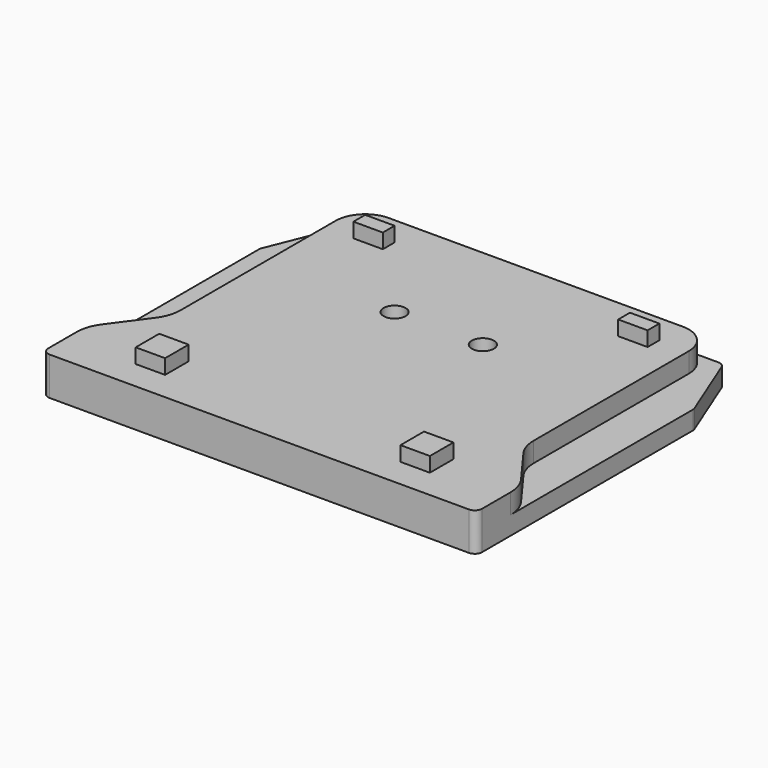
from build123d import *

# Parameters (mm, degrees)
F1_DEPTH      = 2.5
F3_DEPTH      = 2.7
F4_R          = 1
F5_R          = 5
F6_W          = 4
F6_H          = 2
F6_H_2        = 4
F7_DEPTH      = 2
F8_R          = 1.5
F9_DEPTH      = 6
F10_R         = 2.5
F11_DEPTH     = 2.5
F12_S5_R      = 1.5
F12_T6_DEPTH  = 5
F12_S11_R     = 1.5
F12_T12_DEPTH = 5


# Not quite as in the source:
# - a fillet or chamfer that OpenCascade refuses, or shapes differently, is made with other operations: its cross-section is extruded or revolved along the edge and cut away or added


with BuildPart() as f1:
    # F0 (on Top) → F1 (new body)
    with BuildSketch(Plane.XY):
        Polygon((55, 0), (4, 0), (0, -10), (0, -47), (59, -47), (59, -10), align=None)
    extrude(amount=F1_DEPTH)

    # F2 (on face) → F3 (join)
    with BuildSketch(Plane.XY.offset(2.5)):
        with BuildLine():
            Line((0, -39.5), (0, -47))
            Line((0, -47), (59, -47))
            Line((59, -47), (59, -39.5))
            Line((59, -39.5), (53.5, -32))
            Line((53.5, -32), (53.5, -4))
            ThreePointArc((53.5, -4), (52.3284271247, -1.1715728753), (49.5, 0))
            Line((49.5, 0), (9.5, 0))
            ThreePointArc((9.5, 0), (6.6715728753, -1.1715728753), (5.5, -4))
            Line((5.5, -4), (5.5, -32))
            Line((5.5, -32), (0, -39.5))
        make_face()
    extrude(amount=F3_DEPTH)

    # F4
    f4_edges = [f1.edges().sort_by_distance(p)[0] for p in [
        (0, -47, 2.6),
        (59, -47, 2.6),
        (4, 0, 1.25),
        (55, 0, 1.25),
        (59, -10, 1.25),
        (0, -10, 1.25),
    ]]
    fillet(f4_edges, radius=F4_R)

    # F5
    f5_edges = [f1.edges().sort_by_distance(p)[0] for p in [
        (0, -39.5, 3.85),
        (59, -39.5, 3.85),
        (53.5, -32, 3.85),
        (5.5, -32, 3.85),
    ]]
    fillet(f5_edges, radius=F5_R)

    # F6 (on face) → F7 (join)
    with BuildSketch(Plane.XY.offset(5.2)):
        with Locations((11.5, -5)):
            Rectangle(F6_W, F6_H)
        with Locations((11.5, -41)):
            Rectangle(F6_W, F6_H_2)
        with Locations((47.5, -5)):
            Rectangle(F6_W, F6_H)
        with Locations((47.5, -41)):
            Rectangle(F6_W, F6_H_2)
    extrude(amount=F7_DEPTH)

    # F8 (on face) → F9 (cut)
    with BuildSketch(Plane.XY.offset(5.2)):
        with Locations((23.5, -16.5)):
            Circle(F8_R)
        with Locations((35.5, -16.5)):
            Circle(F8_R)
    extrude(amount=-F9_DEPTH, mode=Mode.SUBTRACT)

    # F10 (on face) → F11 (cut)
    with BuildSketch(Plane.XY):
        with Locations((35.5, -16.5)):
            Circle(F10_R)
        with Locations((23.5, -16.5)):
            Circle(F10_R)
    extrude(amount=F11_DEPTH, mode=Mode.SUBTRACT)

    # F12: chamfer of 1.2 on 2 edges, made by hand


with BuildPart() as f12_tool2:
    # F12_s3 → F12_t4 (revolve)
    with BuildSketch(Plane.XZ.offset(16.5)):
        Polygon((38, 1.3), (36.8, 2.5), (38, 2.5), align=None)
    revolve(axis=Axis((35.5, -16.5, 2.5), (0, 0, 1)))

    # F12_s5 → F12_t6 (cut, symmetric)
    with BuildSketch(Plane.XY.offset(1.9)):
        with Locations((35.5, -16.5)):
            Circle(F12_S5_R)
    extrude(amount=F12_T6_DEPTH, both=True, mode=Mode.SUBTRACT)


with BuildPart() as f1_1:
    add(f1.part)

    # F12_t1: union F12_tool2
    add(f12_tool2.part)


with BuildPart() as f12_tool8:
    # F12_s9 → F12_t10 (revolve)
    with BuildSketch(Plane.XZ.offset(16.5)):
        Polygon((26, 1.3), (24.8, 2.5), (26, 2.5), align=None)
    revolve(axis=Axis((23.5, -16.5, 2.5), (0, 0, 1)))

    # F12_s11 → F12_t12 (cut, symmetric)
    with BuildSketch(Plane.XY.offset(1.9)):
        with Locations((23.5, -16.5)):
            Circle(F12_S11_R)
    extrude(amount=F12_T12_DEPTH, both=True, mode=Mode.SUBTRACT)


with BuildPart() as f1_2:
    add(f1_1.part)

    # F12_t7: union F12_tool8
    add(f12_tool8.part)


solid = f1_2.part
